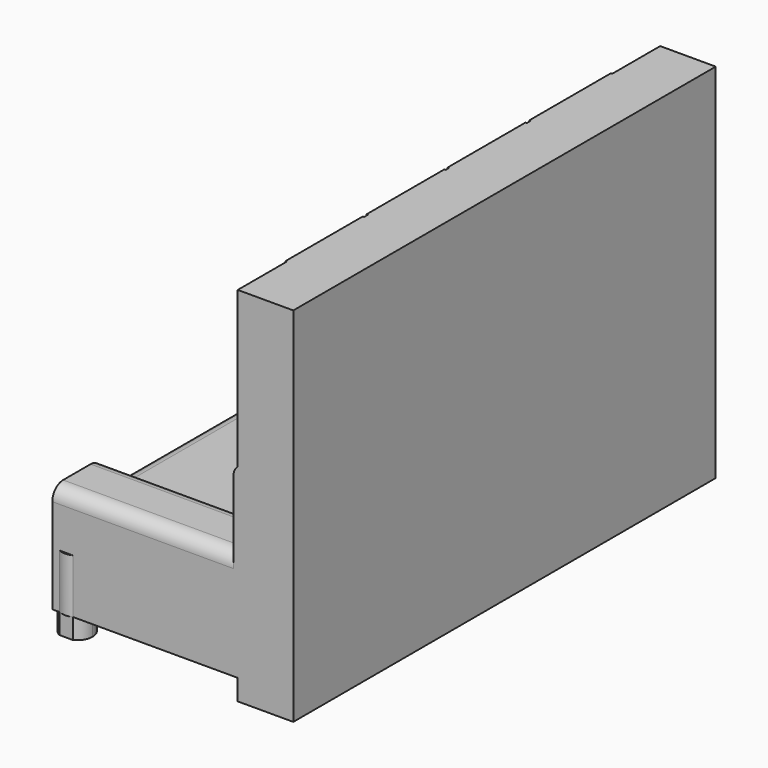
from build123d import *

# Parameters (mm, degrees)
F0_W          = 22.5927522406
F0_H          = 49.5025906712
F1_DEPTH      = 10.16
F2_DEPTH      = 3.81
F3_W          = 11.2244246993
F3_H          = 99.0051813424
F4_DEPTH      = 25.4
F6_DEPTH      = 10.16
F7_R          = 2.54
F8_W          = 33.9610797819
F8_H          = 38.1342638284
F8_H_2        = 37.1269418392
F9_DEPTH      = 5.842
F10_R         = 2.54
F11_W         = 99.0051813424
F11_H         = 67.9221570026
F12_DEPTH     = 10.414
F13_W         = 38.620619569
F13_H         = 17.018
F13_W_2       = 37.6479080878
F14_DEPTH     = 3.302
F15_T1_DEPTH  = 88.9685276568
F15_T6_DEPTH  = 27.94
F15_T11_DEPTH = 27.94
F16_W         = 1.1473407503
F16_H         = 14.478
F17_DEPTH     = 3.302
F18_W         = 19.139082171
F18_H         = 29.1566260799
F18_W_2       = 6.5123029053
F18_H_2       = 0.8140355349
F18_W_3       = 18.2694643736
F18_W_4       = 7.5298482552
F18_W_5       = 18.2365168585
F18_W_6       = 7.1228295565
F18_W_7       = 18.1018151343
F18_W_8       = 7.1228314191
F19_DEPTH     = 0.254
F20_DEPTH     = 1.524


# Not quite as in the source:
# - a fillet or chamfer that OpenCascade refuses, or shapes differently, is made with other operations: its cross-section is extruded or revolved along the edge and cut away or added
# - a feature names something its author has since deleted; it is built from what else it names


with BuildPart() as f1:
    # F0 (on Top) → F1 (new body)
    with BuildSketch(Plane.XY):
        with BuildLine():
            Line((-35.3594812499, 51.6611337662), (-36.6952344775, 51.6611337662))
            Line((-36.6952344775, 51.6611337662), (-36.6952344775, 50.3253805386))
            ThreePointArc((-36.6952344775, 50.3253805386), (-36.1400711383, 51.105970427), (-35.3594812499, 51.6611337662))
        make_face()
        with BuildLine():
            ThreePointArc((-32.8504798068, 51.6611337662), (-34.1049805284, 51.9489325583), (-35.3594812499, 51.6611337662))
            Line((-35.3594812499, 51.6611337662), (-32.8504798068, 51.6611337662))
        make_face()
        with BuildLine():
            Line((-32.8504798068, 51.6611337662), (-35.3594812499, 51.6611337662))
            ThreePointArc((-35.3594812499, 51.6611337662), (-36.1400711383, 51.105970427), (-36.6952344775, 50.3253805386))
            Line((-36.6952344775, 50.3253805386), (-36.6952344775, 47.8163790954))
            ThreePointArc((-36.6952344775, 47.8163790954), (-33.4614356183, 46.2656993361), (-31.2269277871, 49.070879817))
            ThreePointArc((-31.2269277871, 49.070879817), (-31.6663634179, 50.5993869876), (-32.8504798068, 51.6611337662))
        make_face()
        with BuildLine():
            Line((-36.6952344775, 47.8163790954), (-36.6952344775, 50.3253805386))
            ThreePointArc((-36.6952344775, 50.3253805386), (-36.9830332696, 49.070879817), (-36.6952344775, 47.8163790954))
        make_face()
        with BuildLine():
            Line((-14.1024822369, 51.6611337662), (-32.8504798068, 51.6611337662))
            ThreePointArc((-32.8504798068, 51.6611337662), (-31.6663634179, 50.5993869876), (-31.2269277871, 49.070879817))
            ThreePointArc((-31.2269277871, 49.070879817), (-33.4614356183, 46.2656993361), (-36.6952344775, 47.8163790954))
            Line((-36.6952344775, 47.8163790954), (-36.6952344775, 2.158543095))
            Line((-36.6952344775, 2.158543095), (-14.1024822369, 2.158543095))
            Line((-14.1024822369, 2.158543095), (-14.1024822369, 51.6611337662))
        make_face()
        with Locations((-2.8061061166, 26.9098384306)):
            Rectangle(F0_W, F0_H)
        with BuildLine():
            Line((-14.1024822369, 2.158543095), (-36.6952344775, 2.158543095))
            Line((-36.6952344775, 2.158543095), (-36.6952344775, -43.4992929054))
            ThreePointArc((-36.6952344775, -43.4992929054), (-33.4614356183, -41.9486131461), (-31.2269277871, -44.753793627))
            ThreePointArc((-31.2269277871, -44.753793627), (-31.6663634179, -46.2823007976), (-32.8504798068, -47.3440475762))
            Line((-32.8504798068, -47.3440475762), (-14.1024822369, -47.3440475762))
            Line((-14.1024822369, -47.3440475762), (-14.1024822369, 2.158543095))
        make_face()
        with Locations((-2.8061061166, -22.5927522406)):
            Rectangle(F0_W, F0_H)
        with BuildLine():
            ThreePointArc((-31.2269277871, -44.753793627), (-33.4614356183, -41.9486131461), (-36.6952344775, -43.4992929054))
            Line((-36.6952344775, -43.4992929054), (-36.6952344775, -46.0082943486))
            ThreePointArc((-36.6952344775, -46.0082943486), (-36.1400711383, -46.788884237), (-35.3594812499, -47.3440475762))
            Line((-35.3594812499, -47.3440475762), (-32.8504798068, -47.3440475762))
            ThreePointArc((-32.8504798068, -47.3440475762), (-31.6663634179, -46.2823007976), (-31.2269277871, -44.753793627))
        make_face()
        with BuildLine():
            Line((-36.6952344775, -46.0082943486), (-36.6952344775, -43.4992929054))
            ThreePointArc((-36.6952344775, -43.4992929054), (-36.9830332696, -44.753793627), (-36.6952344775, -46.0082943486))
        make_face()
        with BuildLine():
            ThreePointArc((-35.3594812499, -47.3440475762), (-36.1400711383, -46.788884237), (-36.6952344775, -46.0082943486))
            Line((-36.6952344775, -46.0082943486), (-36.6952344775, -47.3440475762))
            Line((-36.6952344775, -47.3440475762), (-35.3594812499, -47.3440475762))
        make_face()
        with BuildLine():
            ThreePointArc((-35.3594812499, -47.3440475762), (-34.1049805284, -47.6318463683), (-32.8504798068, -47.3440475762))
            Line((-32.8504798068, -47.3440475762), (-35.3594812499, -47.3440475762))
        make_face()
    extrude(amount=F1_DEPTH)

    # F0 (on Top) → F2 (join)
    with BuildSketch(Plane.XY):
        with BuildLine():
            Line((-32.8504798068, 51.6611337662), (-35.3594812499, 51.6611337662))
            ThreePointArc((-35.3594812499, 51.6611337662), (-36.1400711383, 51.105970427), (-36.6952344775, 50.3253805386))
            Line((-36.6952344775, 50.3253805386), (-36.6952344775, 47.8163790954))
            ThreePointArc((-36.6952344775, 47.8163790954), (-33.4614356183, 46.2656993361), (-31.2269277871, 49.070879817))
            ThreePointArc((-31.2269277871, 49.070879817), (-31.6663634179, 50.5993869876), (-32.8504798068, 51.6611337662))
        make_face()
        with BuildLine():
            ThreePointArc((-31.2269277871, -44.753793627), (-33.4614356183, -41.9486131461), (-36.6952344775, -43.4992929054))
            Line((-36.6952344775, -43.4992929054), (-36.6952344775, -46.0082943486))
            ThreePointArc((-36.6952344775, -46.0082943486), (-36.1400711383, -46.788884237), (-35.3594812499, -47.3440475762))
            Line((-35.3594812499, -47.3440475762), (-32.8504798068, -47.3440475762))
            ThreePointArc((-32.8504798068, -47.3440475762), (-31.6663634179, -46.2823007976), (-31.2269277871, -44.753793627))
        make_face()
    extrude(amount=-F2_DEPTH)

    # F3 (on face) → F4 (join)
    with BuildSketch(Plane.XY.offset(10.16)):
        with Locations((2.878057654, 2.158543095)):
            Rectangle(F3_W, F3_H)
    extrude(amount=F4_DEPTH)

    # F5 (on face) → F6 (join)
    with BuildSketch(Plane.XY.offset(10.16)):
        Polygon((-2.7341546956, 40.4367111623), (-2.7341546956, 51.6611337662), (-32.8504798068, 51.6611337662), (-35.3594812499, 51.6611337662), (-36.6952344775, 51.6611337662), (-36.6952344775, 50.3253805386), (-36.6952344775, 47.8163790954), (-36.6952344775, 40.4367111623), align=None)
        Polygon((-2.7341546956, -47.3440475762), (-2.7341546956, -35.8318164945), (-36.6952344775, -35.8318164945), (-36.6952344775, -43.4992929054), (-36.6952344775, -46.0082943486), (-36.6952344775, -47.3440475762), (-35.3594812499, -47.3440475762), (-32.8504798068, -47.3440475762), align=None)
    extrude(amount=F6_DEPTH)

    # F7
    f7_edges = [f1.edges().sort_by_distance(p)[0] for p in [
        (-2.734155, 2.158543, 35.56),
        (-19.714695, -35.831816, 20.32),
        (-19.714695, -47.344048, 20.32),
        (-19.714695, 51.661134, 20.32),
        (-19.714695, 40.436711, 20.32),
    ]]
    fillet(f7_edges, radius=F7_R)

    # F8 (on face) → F9 (join)
    with BuildSketch(Plane.XY.offset(10.16)):
        with Locations((-19.7146945866, 21.3695792481)):
            Rectangle(F8_W, F8_H)
        with Locations((-19.7146945866, -17.2683455748)):
            Rectangle(F8_W, F8_H_2)
    extrude(amount=F9_DEPTH)

    # F10
    f10_edges = [f1.edges().sort_by_distance(p)[0] for p in [
        (-19.714695, 1.295125, 16.002),
        (-19.714695, 2.302447, 16.002),
        (-36.695234, -17.268346, 16.002),
        (-36.695234, 21.369579, 16.002),
    ]]
    fillet(f10_edges, radius=F10_R)

    # F11 (on face) → F12 (join)
    with BuildSketch(Plane.YZ.offset(8.4902700037)):
        with Locations((2.158543095, 30.0757006044)):
            Rectangle(F11_W, F11_H)
    extrude(amount=-F12_DEPTH)

    # F13 (on face) → F14 (join)
    with BuildSketch(Plane(origin=(-2.7341546956, 0, 0), x_dir=(0, -1, 0), z_dir=(-1, 0, 0))):
        with Locations((-21.1264013778, 24.511)):
            Rectangle(F13_W, F13_H)
        with Locations((17.0078624506, 24.511)):
            Rectangle(F13_W_2, F13_H)
    extrude(amount=F14_DEPTH)

    # F15: fillet of radius 2.54 on 3 edges, made by hand

    # F15_s2 → F15_t1 (cut)
    with BuildSketch(Plane.XZ.offset(-46.7867111623)):
        with BuildLine():
            ThreePointArc((-6.0361546956, 30.48), (-5.2922059199, 32.2760512242), (-3.4961546956, 33.02))
            Line((-3.4961546956, 33.02), (-6.0361546956, 33.02))
            Line((-6.0361546956, 33.02), (-6.0361546956, 30.48))
        make_face()
    extrude(amount=F15_T1_DEPTH, mode=Mode.SUBTRACT)


with BuildPart() as f15_tool4:
    # F15_s5 → F15_t6 (new body)
    with BuildSketch(Plane.XY.offset(39.37)):
        with BuildLine():
            ThreePointArc((-6.0361546956, 37.8967111623), (-5.2922059199, 39.6927623865), (-3.4961546956, 40.4367111623))
            Line((-3.4961546956, 40.4367111623), (-6.0361546956, 40.4367111623))
            Line((-6.0361546956, 40.4367111623), (-6.0361546956, 37.8967111623))
        make_face()
    extrude(amount=-F15_T6_DEPTH)

    split(bisect_by=Plane.XY.offset(16.002), keep=Keep.TOP)


with BuildPart() as f1_1:
    add(f1.part)

    # F15_t3: cut F15_tool4
    add(f15_tool4.part, mode=Mode.SUBTRACT)


with BuildPart() as f15_tool9:
    # F15_s10 → F15_t11 (new body)
    with BuildSketch(Plane.XY.offset(11.43)):
        with BuildLine():
            ThreePointArc((-6.0361546956, -33.2918164945), (-5.2922059199, -35.0878677187), (-3.4961546956, -35.8318164945))
            Line((-3.4961546956, -35.8318164945), (-6.0361546956, -35.8318164945))
            Line((-6.0361546956, -35.8318164945), (-6.0361546956, -33.2918164945))
        make_face()
    extrude(amount=F15_T11_DEPTH)

    split(bisect_by=Plane.XY.offset(16.002), keep=Keep.TOP)


with BuildPart() as f1_2:
    add(f1_1.part)

    # F15_t8: cut F15_tool9
    add(f15_tool9.part, mode=Mode.SUBTRACT)

    # F16 (on face) → F17 (cut)
    with BuildSketch(Plane(origin=(-6.0361546956, 0, 0), x_dir=(0, -1, 0), z_dir=(-1, 0, 0))):
        with Locations((-1.7287769588, 23.241)):
            Rectangle(F16_W, F16_H)
    extrude(amount=-F17_DEPTH, mode=Mode.SUBTRACT)

    # F18 (on face) → F19 (join)
    with BuildSketch(Plane(origin=(-1.9237299963, 0, 0), x_dir=(0, -1, 0), z_dir=(-1, 0, 0))):
        with Locations((-30.8671663515, 49.4584660657)):
            Rectangle(F18_W, F18_H)
        with Locations((-30.3225759417, 61.080571264)):
            Rectangle(F18_W_2, F18_H_2, mode=Mode.SUBTRACT)
        with Locations((-11.2932752818, 49.4584660657)):
            Rectangle(F18_W_3, F18_H)
        with Locations((-11.4979553036, 61.080571264)):
            Rectangle(F18_W_4, F18_H_2, mode=Mode.SUBTRACT)
        with Locations((7.7183801332, 49.4584660657)):
            Rectangle(F18_W_5, F18_H)
        with Locations((7.9371919855, 61.080571264)):
            Rectangle(F18_W_6, F18_H_2, mode=Mode.SUBTRACT)
        with Locations((26.7809126526, 49.4584660657)):
            Rectangle(F18_W_7, F18_H)
        with Locations((27.0670773461, 61.080571264)):
            Rectangle(F18_W_8, F18_H_2, mode=Mode.SUBTRACT)
    extrude(amount=F19_DEPTH)

    # F18 (on face) → F20 (join)
    with BuildSketch(Plane(origin=(-1.9237299963, 0, 0), x_dir=(0, -1, 0), z_dir=(-1, 0, 0))):
        with Locations((27.0670773461, 61.080571264)):
            Rectangle(F18_W_8, F18_H_2)
        with Locations((7.9371919855, 61.080571264)):
            Rectangle(F18_W_6, F18_H_2)
        with Locations((-11.4979553036, 61.080571264)):
            Rectangle(F18_W_4, F18_H_2)
        with Locations((-30.3225759417, 61.080571264)):
            Rectangle(F18_W_2, F18_H_2)
    extrude(amount=F20_DEPTH)


solid = f1_2.part
